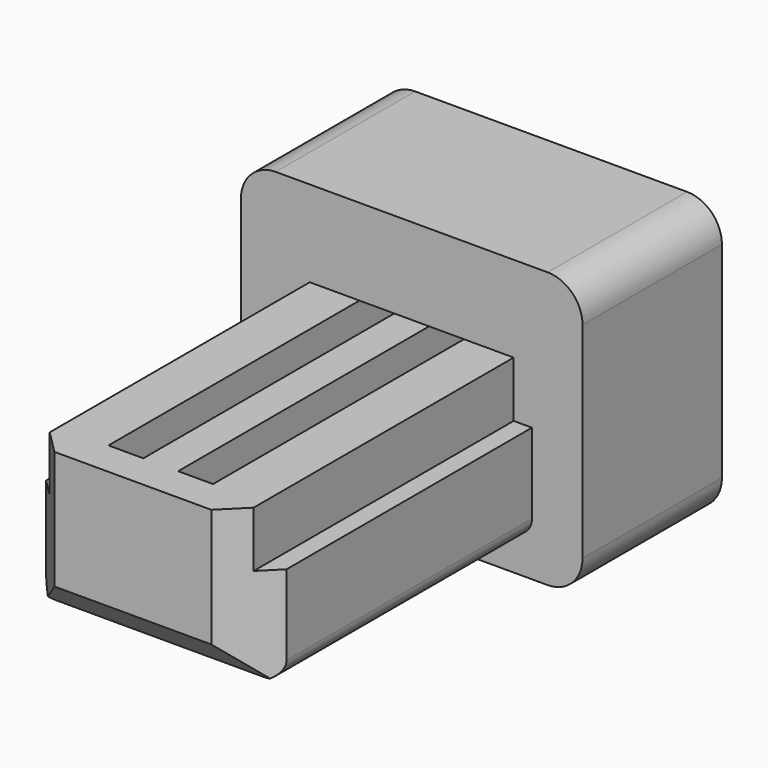
from build123d import *

# Parameters (mm, degrees)
F1_DEPTH    = 10
F2_SIZE     = 1.2
F3_R        = 0.5
F5_W        = 9.8
F5_H        = 7.9
F6_DEPTH    = 5
F8_DEPTH    = 2.2
F9_T1_DEPTH = 9.6433659759
F10_R       = 1


# Not quite as in the source:
# - a fillet or chamfer that OpenCascade refuses, or shapes differently, is made with other operations: its cross-section is extruded or revolved along the edge and cut away or added


with BuildPart() as f1:
    # F0 (on Front) → F1 (new body)
    with BuildSketch(Plane.XZ):
        Polygon((-3.45, 2.8), (-3.45, 0), (3.45, 0), (3.45, 2.8), (2.925, 2.8), (2.925, 4.4), (-2.925, 4.4), (-2.925, 2.8), align=None)
    extrude(amount=F1_DEPTH)

    # F2
    f2_edges = [f1.edges().sort_by_distance(p)[0] for p in [
        (3.45, -10, 1.4),
        (-3.45, -10, 1.4),
    ]]
    chamfer(f2_edges, length=F2_SIZE)

    # F3
    f3_edges = [f1.edges().sort_by_distance(p)[0] for p in [
        (-3.45, -4.4, 0),
        (3.45, -4.4, 0),
    ]]
    fillet(f3_edges, radius=F3_R)

    # F5 (on Front) → F6 (join)
    with BuildSketch(Plane.XZ):
        with Locations((0, 2.92)):
            Rectangle(F5_W, F5_H)
    extrude(amount=-F6_DEPTH)

    # F7 (on offset) → F8 (cut)
    with BuildSketch(Plane.XY.offset(4.4)):
        Polygon((-1.5, 0), (-1.5, -9), (-0.5, -9), (-0.5, 5), (-1.5, 5), align=None)
        Polygon((1.5, 5), (0.5, 5), (0.5, -9), (1.5, -9), (1.5, 0), align=None)
    extrude(amount=-F8_DEPTH, mode=Mode.SUBTRACT)

    # F9: chamfer of 1 on 1 edges, made by hand

    # F9_s2 → F9_t1 (cut)
    with BuildSketch(Plane.YZ.offset(-4.821682988)):
        Polygon((-9, 0), (-10, 1), (-10, 0), align=None)
    extrude(amount=F9_T1_DEPTH, mode=Mode.SUBTRACT)

    # F10
    f10_edges = [f1.edges().sort_by_distance(p)[0] for p in [
        (4.9, 2.5, 6.87),
        (4.9, 2.5, -1.03),
        (-4.9, 2.5, -1.03),
        (-4.9, 2.5, 6.87),
    ]]
    fillet(f10_edges, radius=F10_R)


solid = f1.part
